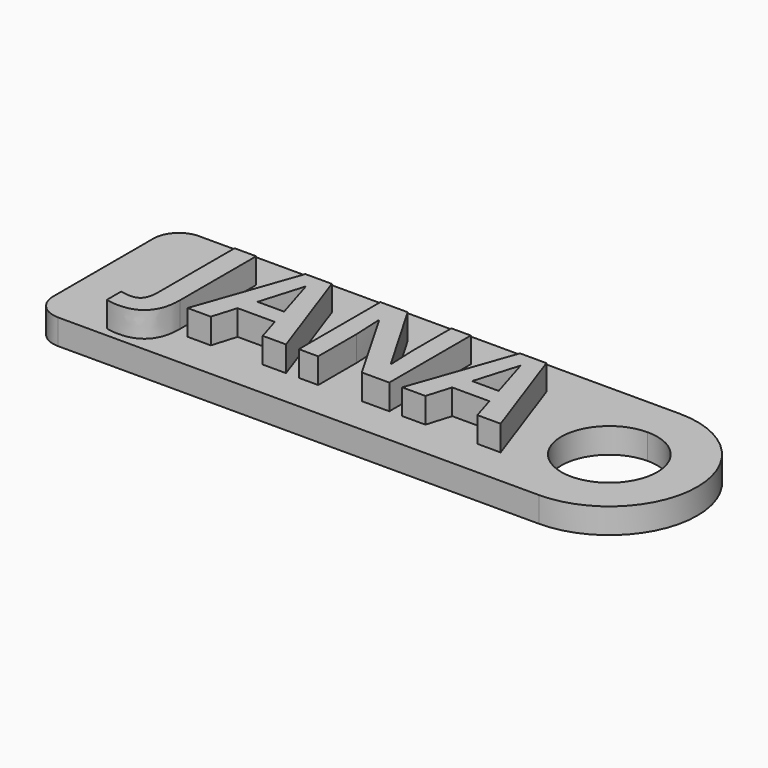
from build123d import *

# Parameters (mm, degrees)
F1_DEPTH     = 2
F2_R         = 2
F3_TEXT_SIZE = 11.2880351177
F4_DEPTH     = 2


# Not quite as in the source:
# - Text() gives the source's letters only with a copy of the font that has no kerning and outlines rounded to 1/6400 em; it was checked with that copy


with BuildPart() as f1:
    # F0 (on Top) → F1 (new body)
    with BuildSketch(Plane.XY):
        with BuildLine():
            Line((20, 6.9603520454), (-20, 6.9603520454))
            Line((-20, 6.9603520454), (-20, -6.9603520454))
            Line((-20, -6.9603520454), (20, -6.9603520454))
            Line((20, -6.9603520454), (20, -3.7914942375))
            ThreePointArc((20, -3.7914942375), (16.2085057625, 0), (20, 3.7914942375))
            Line((20, 3.7914942375), (20, 6.9603520454))
        make_face()
        with BuildLine():
            ThreePointArc((20, -6.9603520454), (26.9603520454, 0), (20, 6.9603520454))
            Line((20, 6.9603520454), (20, 3.7914942375))
            ThreePointArc((20, 3.7914942375), (22.6809912862, 2.6809912862), (23.7914942375, 0))
            ThreePointArc((23.7914942375, 0), (22.6809912862, -2.6809912862), (20, -3.7914942375))
            Line((20, -3.7914942375), (20, -6.9603520454))
        make_face()
    extrude(amount=F1_DEPTH)

    # F2
    f2_edges = [f1.edges().sort_by_distance(p)[0] for p in [
        (-20, 6.960352, 1),
        (-20, -6.960352, 1),
    ]]
    fillet(f2_edges, radius=F2_R)

    # F3 (on face) → F4 (join)
    with BuildSketch(Plane.XY.offset(2)):
        with Locations((-13.8914212584, -3.9901267737)):
            Text('JANA', F3_TEXT_SIZE, font='Open Sans', font_style=FontStyle.BOLD, text_align=(TextAlign.LEFT, TextAlign.BOTTOM))
    extrude(amount=F4_DEPTH)


solid = f1.part
